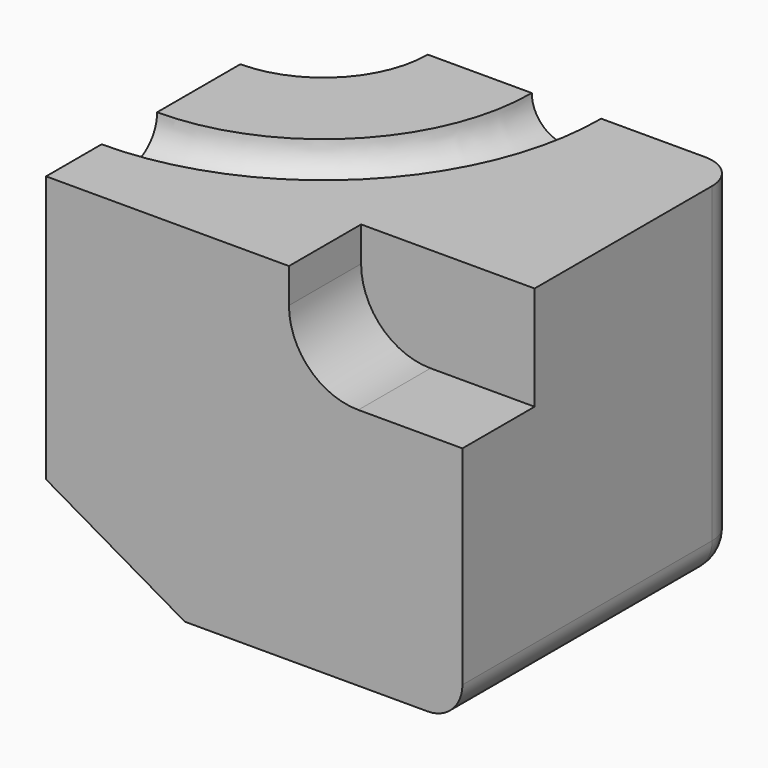
from build123d import *

# Parameters (mm, degrees)
F0_W        = 60
F0_H        = 50
F1_DEPTH    = 50
F2_W        = 15
F2_H        = 50
F5_DEPTH    = 13
F6_T1_DEPTH = 138.4834301858
F7_R        = 5


# Not quite as in the source:
# - a fillet or chamfer that OpenCascade refuses, or shapes differently, is made with other operations: its cross-section is extruded or revolved along the edge and cut away or added


with BuildPart() as f1:
    # F0 (on Top) → F1 (new body)
    with BuildSketch(Plane.XY):
        with Locations((30, -25)):
            Rectangle(F0_W, F0_H)
    extrude(amount=F1_DEPTH)

    # F2 (on Right) → F3 (revolve, cut)
    with BuildSketch(Plane.YZ):
        with Locations((-7.5, 25)):
            Rectangle(F2_W, F2_H)
        with BuildLine():
            Line((-30, 50), (-40, 50))
            ThreePointArc((-40, 50), (-35, 45), (-30, 50))
        make_face()
    revolve(axis=Axis((0, 0, 25), (0, 0, 1)), mode=Mode.SUBTRACT)

    # F4 (on face) → F5 (cut)
    with BuildSketch(Plane.XZ.offset(50)):
        with BuildLine():
            Line((60, 50), (35, 50))
            Line((35, 50), (35, 45))
            ThreePointArc((35, 45), (37.9289321881, 37.9289321881), (45, 35))
            Line((45, 35), (60, 35))
            Line((60, 35), (60, 50))
        make_face()
    extrude(amount=-F5_DEPTH, mode=Mode.SUBTRACT)

    # F6: chamfer of 20 x 11.5470053838 on 1 edges, made by hand

    # F6_s2 → F6_t1 (cut)
    with BuildSketch(Plane.XZ.offset(-36.7417150929)):
        Polygon((20, 0), (0, 11.5470053838), (0, 0), align=None)
    extrude(amount=F6_T1_DEPTH, mode=Mode.SUBTRACT)

    # F7
    f7_edges = [f1.edges().sort_by_distance(p)[0] for p in [
        (60, 0, 25),
        (60, -25, 0),
        (40, 0, 0),
    ]]
    fillet(f7_edges, radius=F7_R)


solid = f1.part
